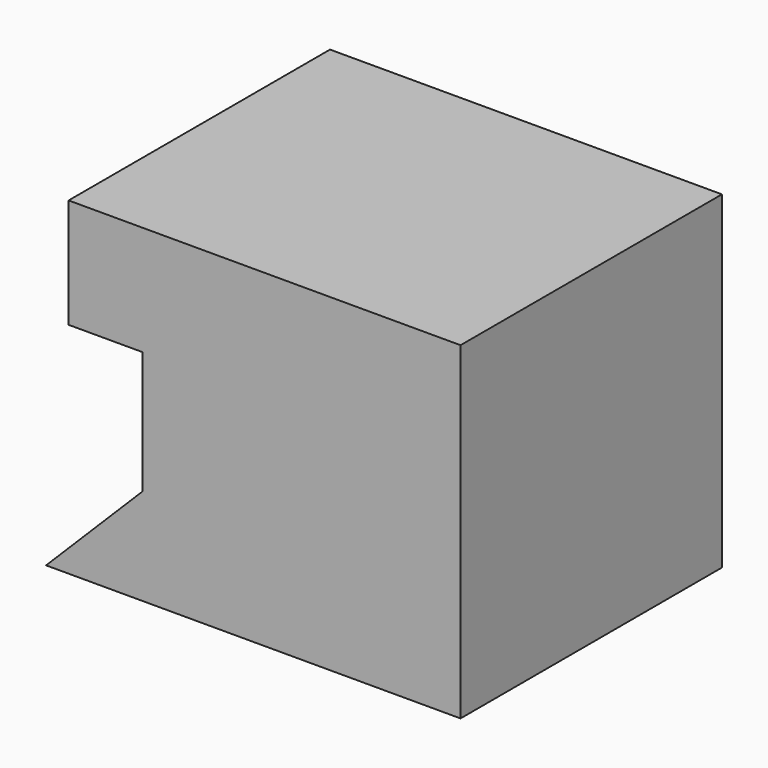
from build123d import *

# Parameters (mm, degrees)
F0_W        = 109.5967777073
F0_H        = 74.5766162872
F1_DEPTH    = 25
F2_W        = 72.5555187091
F2_H        = 74.5766162872
F3_DEPTH    = 25
F4_W        = 72.5555187091
F4_H        = 74.5766162872
F4_W_2      = 16.8990129605
F5_DEPTH    = 25
F6_T4_DEPTH = 280.3112553245


# Not quite as in the source:
# - a fillet or chamfer that OpenCascade refuses, or shapes differently, is made with other operations: its cross-section is extruded or revolved along the edge and cut away or added


with BuildPart() as f1:
    # F0 (on Top) → F1 (new body)
    with BuildSketch(Plane.XY):
        with Locations((3.1754020602, -3.2661296427)):
            Rectangle(F0_W, F0_H)
    extrude(amount=F1_DEPTH)

    # F2 (on face) → F3 (join)
    with BuildSketch(Plane.XY.offset(25)):
        with Locations((21.6960315593, -3.2661296427)):
            Rectangle(F2_W, F2_H)
    extrude(amount=F3_DEPTH)

    # F4 (on face) → F5 (join)
    with BuildSketch(Plane.XY.offset(50)):
        with Locations((21.6960315593, -3.2661296427)):
            Rectangle(F4_W, F4_H)
        with Locations((-23.0312342755, -3.2661296427)):
            Rectangle(F4_W_2, F4_H)
    extrude(amount=F5_DEPTH)

    # F6: chamfer of 40 on 1 edges, made by hand


with BuildPart() as f6_tool2:
    # F6_s3 → F6_t4 (new body)
    with BuildSketch(Plane.XZ.offset(-136.8894980195)):
        Polygon((-51.6229867935, -15), (-11.6229867935, 25), (-51.6229867935, 25), align=None)
    extrude(amount=F6_T4_DEPTH)

    split(bisect_by=Plane.YZ.offset(-14.5817277953), keep=Keep.BOTTOM)


with BuildPart() as f1_1:
    add(f1.part)

    # F6_t1: cut F6_tool2
    add(f6_tool2.part, mode=Mode.SUBTRACT)


solid = f1_1.part
